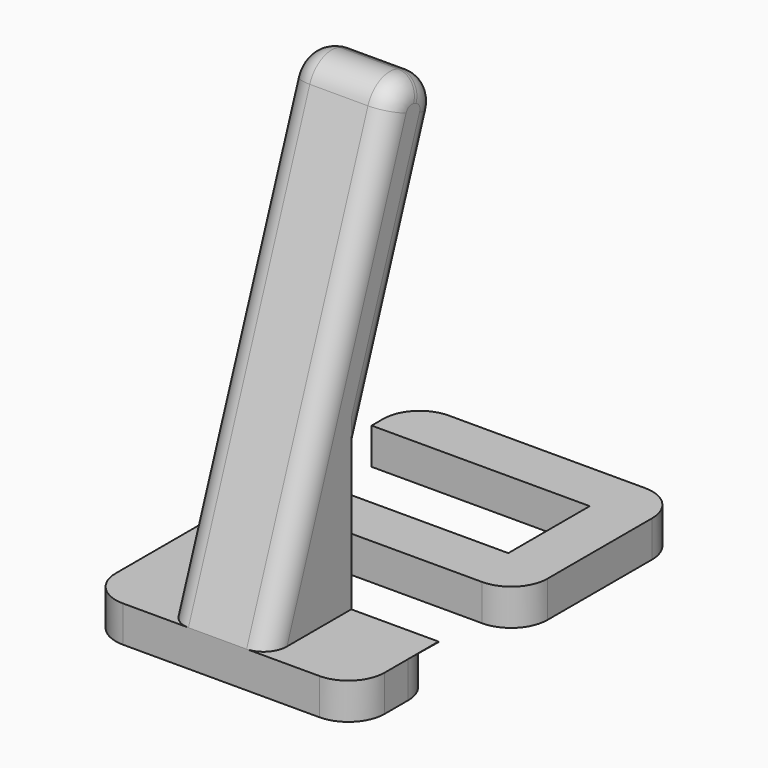
from build123d import *

# Parameters (mm, degrees)
F1_DEPTH = 5
F3_DEPTH = 37
F5_DEPTH = 36.2749
F6_R     = 4
F7_R     = 3
F8_R     = 4.99999


# Not quite as in the source:
# - a fillet or chamfer is up to 0.001 mm smaller than in the source, because OpenCascade refuses the exact size


with BuildPart() as f1:
    # F0 (on Top) → F1 (new body)
    with BuildSketch(Plane.XY):
        Polygon((0, 35), (0, 0), (37, 0), (37, 14), (7, 14), (7, 28), (37, 28), (37, 35), (37, 56), (0, 56), (0, 49), (30, 49), (30, 35), align=None)
    extrude(amount=F1_DEPTH)

    # F2 (on Right) → F3 (join)
    with BuildSketch(Plane.YZ):
        Polygon((22.2313093162, 66.0800203511), (0, 5), (9, 5), (14.2503125495, 4.9267373979), (14.2503125495, 19.4251151749), (30.1785093102, 63.1874761075), align=None)
    extrude(amount=F3_DEPTH)

    # F4 (on Front) → F5 (cut)
    with BuildSketch(Plane.XZ):
        Polygon((11, 5), (11, 66.0800203511), (25, 66.0800203511), (25, 5), (61.9937415394, 5), (61.9937415394, 77.6014764043), (-15.3317964795, 77.6014764043), (-15.3317964795, 5), align=None)
    extrude(amount=-F5_DEPTH, mode=Mode.SUBTRACT)

    # F6
    f6_edges = [f1.edges().sort_by_distance(p)[0] for p in [
        (18, 22.231309, 66.08002),
        (18, 30.178509, 63.187476),
    ]]
    fillet(f6_edges, radius=F6_R)

    # F7
    f7_edges = [f1.edges().sort_by_distance(p)[0] for p in [
        (11, 21.530371, 39.42691),
        (11, 10.431614, 33.660625),
        (25, 21.530371, 39.42691),
        (25, 10.431614, 33.660625),
    ]]
    fillet(f7_edges, radius=F7_R)

    # F8 (radius 5 in the source; OpenCascade refuses exactly that, so slightly less here)
    f8_edges = [f1.edges().sort_by_distance(p)[0] for p in [
        (37, 0, 2.5),
        (37, 28, 2.5),
        (37, 14, 2.465115),
        (0, 0, 2.5),
        (0, 35, 2.5),
        (0, 56, 2.5),
        (37, 56, 2.5),
    ]]
    fillet(f8_edges, radius=F8_R)


solid = f1.part
